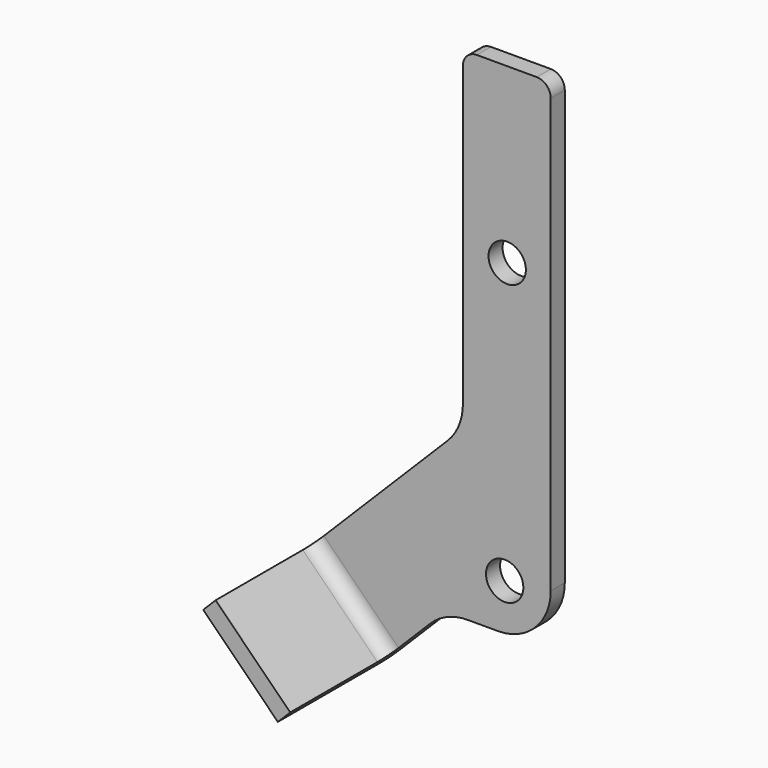
from build123d import *

# Parameters (mm, degrees)
F1_DEPTH = 6.35
F3_DEPTH = 50.8
F5_D     = 13.49248
F6_R     = 19.05
F7_R     = 5.08
F8_R     = 5.08


# Not quite as in the source:
# - a feature names something its author has since deleted; it is built from what else it names


with BuildPart() as f1:
    # F0 (on Front) → F1 (new body)
    with BuildSketch(Plane.XZ):
        Polygon((37.9981123171, 180.8299914), (6.2481123171, 180.8299914), (6.2481123171, 60.2186896705), (-47.5612342455, 6.2650593709), (-20.5844190958, -20.6396139104), (0, 0), (6.2481123171, 0), (37.9981123171, 0), (37.9981123171, 33.02), align=None)
    extrude(amount=F1_DEPTH)

    # F2 (on face) → F3 (join)
    with BuildSketch(Plane(origin=(0, 0, 0), x_dir=(-1, 0, 0), z_dir=(0, 1, 0))):
        Polygon((52.0453464591, 1.7689235126), (47.5612342455, 6.2650593709), (20.5844190958, -20.6396139104), (25.0685313093, -25.1357497687), align=None)
    extrude(amount=-F3_DEPTH)

    # F5 (through all)
    with Locations(Plane.XZ.offset(6.35)):
        with Locations((22.2628123171, 118.2443914), (21.3484123171, 16.8009124652)):
            Hole(F5_D / 2)

    # F6
    f6_edges = [f1.edges().sort_by_distance(p)[0] for p in [
        (6.248112, -3.175, 60.21869),
        (37.998112, -3.175, 0),
        (0, -3.175, 0),
    ]]
    fillet(f6_edges, radius=F6_R)

    # F7
    f7_edges = [f1.edges().sort_by_distance(p)[0] for p in [
        (-38.556939, 0, -11.683413),
        (-34.072827, -6.35, -7.187277),
    ]]
    fillet(f7_edges, radius=F7_R)

    # F8
    f8_edges = [f1.edges().sort_by_distance(p)[0] for p in [
        (6.248112, -3.175, 180.829991),
        (37.998112, -3.175, 180.829991),
    ]]
    fillet(f8_edges, radius=F8_R)


solid = f1.part
